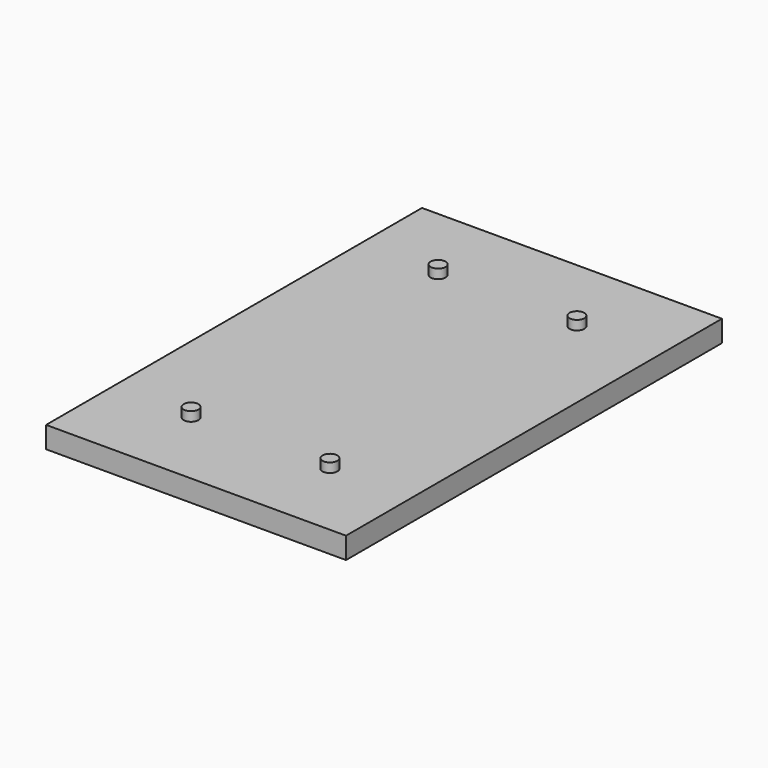
from build123d import *

# Parameters (mm, degrees)
F0_W      = 55.85
F0_H      = 3
F1_DEPTH  = 87.49
F2_T      = -0.75
F3_DEPTH  = 0.75
F4_W      = 20
F4_H      = 7
F4_W_2    = 16
F4_H_2    = 3
F5_DEPTH  = 0.75
F7_ANGLE  = 90
F8_ANGLE  = 90
F10_ANGLE = 90
F11_ANGLE = 90
F12_R     = 1.5
F13_R     = 1.5
F15_ANGLE = 90
F16_DEPTH = 1
F17_R     = 1.5
F18_R     = 1.5
F19_R     = 1.49999
F20_R     = 1.49999
F21_R     = 4
F22_R     = 4
F23_W     = 55.85
F23_H     = 87.49
F24_DEPTH = 4
F25_T     = -0.25
F26_R     = 9.693411876
F27_DEPTH = 0.25
F29_R     = 1.375
F30_DEPTH = 1.74


# Not quite as in the source:
# - a fillet or chamfer is up to 0.001 mm smaller than in the source, because OpenCascade refuses the exact size


with BuildPart() as f1:
    # F0 (on Front) → F1 (new body)
    with BuildSketch(Plane.XZ):
        with Locations((-39.0305130277, -21.5327367023)):
            Rectangle(F0_W, F0_H)
    extrude(amount=-F1_DEPTH)

    # F2
    f2_openings = [f1.faces().sort_by_distance(p)[0] for p in [
        (-39.030513, 43.745, -20.032737),
    ]]
    offset(amount=F2_T, openings=f2_openings)

    # F3 (cut): a face of the model
    f3_faces = [f1.faces().sort_by_distance(p)[0] for p in [
        (-39.0305130277, 86.74, -21.1577367023),
    ]]
    extrude(f3_faces, amount=-F3_DEPTH, mode=Mode.SUBTRACT)

    # F4 (on face) → F5 (join, through all)
    with BuildSketch(Plane.XY.offset(-22.2827367023)):
        with Locations((-39.0305130277, 90.99)):
            Rectangle(F4_W, F4_H)
        with Locations((-39.0305130277, 90.99)):
            Rectangle(F4_W_2, F4_H_2, mode=Mode.SUBTRACT)
    extrude(amount=-F5_DEPTH)

    # F6 (on face) → F7 (revolve)
    with BuildSketch(Plane.YZ.offset(-66.2055130277)):
        with BuildLine():
            Line((82.49, -21.0327367023), (83.365, -21.0327367023))
            ThreePointArc((83.365, -21.0327367023), (82.49, -20.1577367023), (81.615, -21.0327367023))
            Line((81.615, -21.0327367023), (82.49, -21.0327367023))
        make_face()
    revolve(axis=Axis((-66.2055130277, 82.0525, -21.0327367023), (0, 1, 0)), revolution_arc=F7_ANGLE)

    # F6 (on face) → F8 (revolve)
    with BuildSketch(Plane.YZ.offset(-66.2055130277)):
        with BuildLine():
            Line((27.49, -21.0327367023), (28.365, -21.0327367023))
            ThreePointArc((28.365, -21.0327367023), (27.49, -20.1577367023), (26.615, -21.0327367023))
            Line((26.615, -21.0327367023), (27.49, -21.0327367023))
        make_face()
    revolve(axis=Axis((-66.2055130277, 27.0525, -21.0327367023), (0, 1, 0)), revolution_arc=F8_ANGLE)

    # F9 (on face) → F10 (revolve)
    with BuildSketch(Plane(origin=(-11.8555130277, 0, 0), x_dir=(0, -1, 0), z_dir=(-1, 0, 0))):
        with BuildLine():
            Line((-83.365, -21.0327367023), (-81.615, -21.0327367023))
            ThreePointArc((-81.615, -21.0327367023), (-82.49, -20.1577367023), (-83.365, -21.0327367023))
        make_face()
    revolve(axis=Axis((-11.8555130277, 82.49, -21.0327367023), (0, -1, 0)), revolution_arc=F10_ANGLE)

    # F9 (on face) → F11 (revolve)
    with BuildSketch(Plane(origin=(-11.8555130277, 0, 0), x_dir=(0, -1, 0), z_dir=(-1, 0, 0))):
        with BuildLine():
            Line((-28.365, -21.0327367023), (-26.615, -21.0327367023))
            ThreePointArc((-26.615, -21.0327367023), (-27.49, -20.1577367023), (-28.365, -21.0327367023))
        make_face()
    revolve(axis=Axis((-11.8555130277, 27.49, -21.0327367023), (0, -1, 0)), revolution_arc=F11_ANGLE)

    # F12
    f12_edges = [f1.edges().sort_by_distance(p)[0] for p in [
        (-66.205513, 0.75, -21.157737),
    ]]
    fillet(f12_edges, radius=F12_R)

    # F13
    f13_edges = [f1.edges().sort_by_distance(p)[0] for p in [
        (-11.855513, 0.75, -21.157737),
    ]]
    fillet(f13_edges, radius=F13_R)

    # F14 (on face) → F15 (revolve)
    with BuildSketch(Plane(origin=(0, 0.75, 0), x_dir=(-1, 0, 0), z_dir=(0, 1, 0))):
        with BuildLine():
            Line((38.1555130277, -21.0327367023), (39.9055130277, -21.0327367023))
            ThreePointArc((39.9055130277, -21.0327367023), (39.0305130277, -20.1577367023), (38.1555130277, -21.0327367023))
        make_face()
    revolve(axis=Axis((-39.0305130277, 0.75, -21.0327367023), (-1, 0, 0)), revolution_arc=F15_ANGLE)

    # F16 (add): a face of the model
    f16_faces = [f1.faces().sort_by_distance(p)[0] for p in [
        (-39.0305130277, 44.6180943483, -23.0327367023),
    ]]
    extrude(f16_faces, amount=F16_DEPTH)

    # F17
    f17_edges = [f1.edges().sort_by_distance(p)[0] for p in [
        (-47.030513, 89.49, -23.157737),
    ]]
    fillet(f17_edges, radius=F17_R)

    # F18
    f18_edges = [f1.edges().sort_by_distance(p)[0] for p in [
        (-31.030513, 89.49, -23.157737),
    ]]
    fillet(f18_edges, radius=F18_R)

    # F19 (radius 1.5 in the source; OpenCascade refuses exactly that, so slightly less here)
    f19_edges = [f1.edges().sort_by_distance(p)[0] for p in [
        (-31.030513, 92.49, -23.157737),
    ]]
    fillet(f19_edges, radius=F19_R)

    # F20 (radius 1.5 in the source; OpenCascade refuses exactly that, so slightly less here)
    f20_edges = [f1.edges().sort_by_distance(p)[0] for p in [
        (-47.030513, 92.49, -23.157737),
    ]]
    fillet(f20_edges, radius=F20_R)

    # F21
    f21_edges = [f1.edges().sort_by_distance(p)[0] for p in [
        (-29.030513, 94.49, -23.157737),
    ]]
    fillet(f21_edges, radius=F21_R)

    # F22
    f22_edges = [f1.edges().sort_by_distance(p)[0] for p in [
        (-49.030513, 94.49, -23.157737),
    ]]
    fillet(f22_edges, radius=F22_R)


with BuildPart() as f24:
    # F23 (on face) → F24 (new body)
    with BuildSketch(Plane(origin=(0, 0, -24.0327367023), x_dir=(1, 0, 0), z_dir=(0, 0, -1))):
        with Locations((-39.0305130277, -43.745)):
            Rectangle(F23_W, F23_H)
    extrude(amount=F24_DEPTH)

    # F25
    f25_openings = [f24.faces().sort_by_distance(p)[0] for p in [
        (-39.030513, 87.49, -26.032737),
    ]]
    offset(amount=F25_T, openings=f25_openings)

    # F26 (on face) → F27 (cut, through all)
    with BuildSketch(Plane(origin=(0, 0, -28.0327367023), x_dir=(1, 0, 0), z_dir=(0, 0, -1))):
        with Locations((-39.0305130277, -43.745)):
            Circle(F26_R)
    extrude(amount=-F27_DEPTH, mode=Mode.SUBTRACT)

    # F29 (on face) → F30 (join)
    with BuildSketch(Plane.XY.offset(-24.0327367023)):
        with Locations((-51.9555130277, 15)):
            Circle(F29_R)
        with Locations((-26.1055130277, 15)):
            Circle(F29_R)
        with Locations((-26.1055130277, 72.49)):
            Circle(F29_R)
        with Locations((-51.9555130277, 72.49)):
            Circle(F29_R)
    extrude(amount=F30_DEPTH)


solid = f24.part
